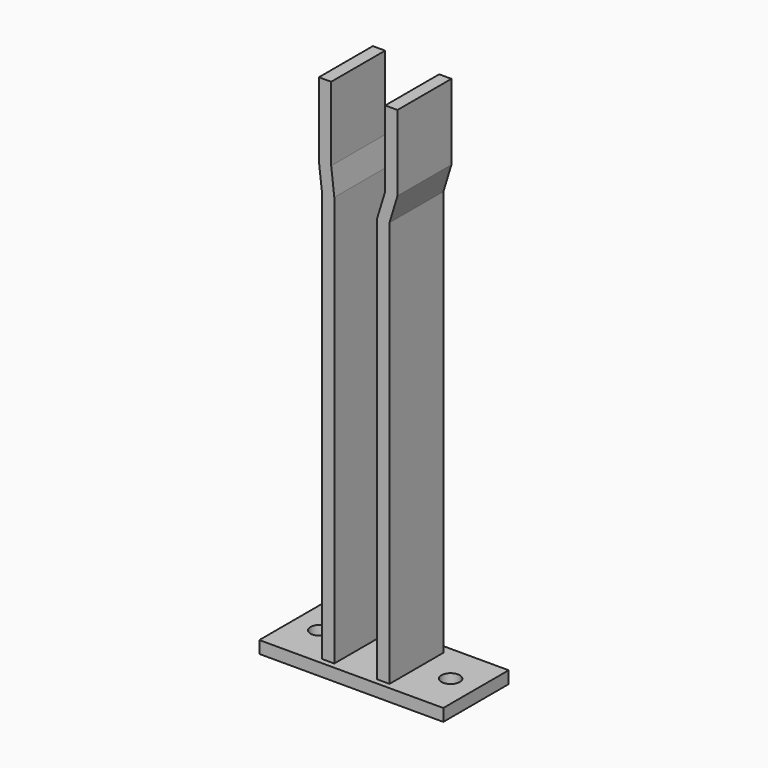
from build123d import *

# Parameters (mm, degrees)
F0_W     = 40
F0_H     = 6
F1_DEPTH = 90
F4_D     = 9
F5_W     = 6
F5_H     = 36.9851887226
F5_H_2   = 204.6339064837
F5_H_3   = 206.7867070436
F5_H_4   = 36.1703634262
F6_DEPTH = 18
F7_DEPTH = 15


# Not quite as in the source:
# - a feature names something its author has since deleted; it is built from what else it names


with BuildPart() as f1:
    # F0 (on Right) → F1 (new body)
    with BuildSketch(Plane.YZ):
        with Locations((-0.72813743, 3)):
            Rectangle(F0_W, F0_H)
    extrude(amount=F1_DEPTH)

    # F4 (through all)
    with Locations(Plane(origin=(0, 0, 0), x_dir=(1, 0, 0), z_dir=(0, 0, -1))):
        with Locations((13, 0), (77, 0)):
            Hole(F4_D / 2)

    # F5 (on Front) → F6 (join)
    with BuildSketch(Plane.XZ):
        with Locations((62.4182647765, 235.9948903322)):
            Rectangle(F5_W, F5_H)
        Polygon((59.4182647765, 217.5022959709), (55.5, 204.6339064837), (61.5, 204.6339064837), (65.4182647765, 217.5022959709), align=None)
        with Locations((58.5, 102.3169532418)):
            Rectangle(F5_W, F5_H_2)
        with Locations((31.5, 103.3933535218)):
            Rectangle(F5_W, F5_H_3)
        Polygon((26.9661769271, 219.9091017246), (28.5, 206.7867070436), (34.5, 206.7867070436), (32.9661769271, 219.9091017246), align=None)
        with Locations((29.9661769271, 237.9942834377)):
            Rectangle(F5_W, F5_H_4)
    extrude(amount=F6_DEPTH)

    # F7 (add): faces of the model
    f7_faces = [f1.faces().sort_by_distance(p)[0] for p in [
        (31.2379126918, 0, 131.0397325754),
        (59.1846567788, 0, 130.2437423468),
    ]]
    extrude(f7_faces, amount=F7_DEPTH)


solid = f1.part
